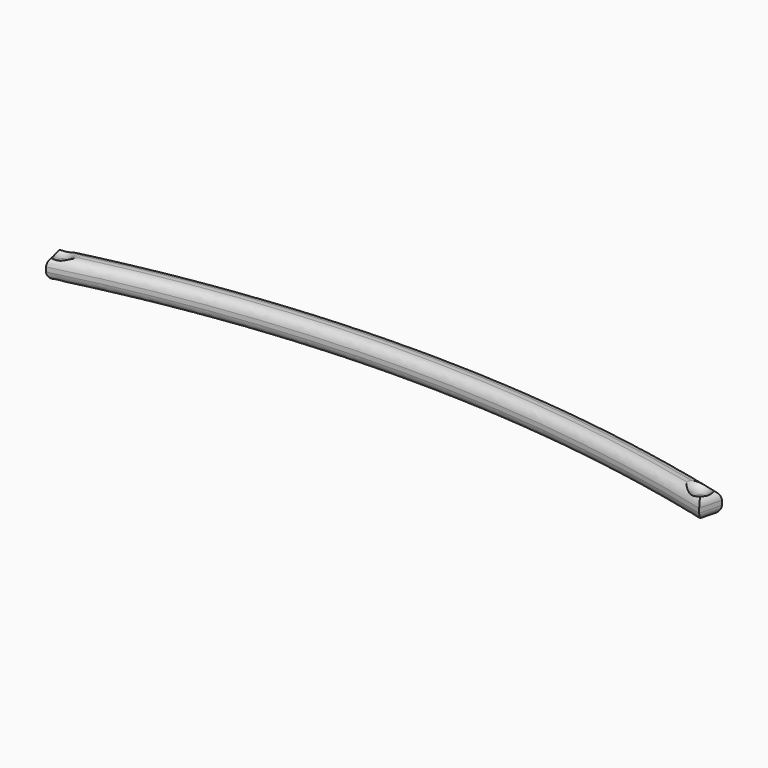
from build123d import *

# Parameters (mm, degrees)
F0_R         = 1.5
F1_DEPTH     = 5
F2_T1_DEPTH  = 15
F2_T3_DEPTH  = 15
F2_T6_ANGLE  = 30.897335
F2_T8_ANGLE  = 30.864963
F2_T14_ANGLE = 30.897335
F2_T16_ANGLE = 30.864963


# Not quite as in the source:
# - a fillet or chamfer that OpenCascade refuses, or shapes differently, is made with other operations: its cross-section is extruded or revolved along the edge and cut away or added


with BuildPart() as f1:
    # F0 (on Top) → F1 (new body)
    with BuildSketch(Plane.XY):
        with BuildLine():
            Line((73.75, -4.841229), (75, 0))
            ThreePointArc((75, 0), (0, 9.526249), (-75, 0))
            Line((-75, 0), (-73.75, -4.841229))
            ThreePointArc((-73.75, -4.841229), (0, 4.526249), (73.75, -4.841229))
        make_face()
        with Locations((-72.566904, -1.807881)):
            Circle(F0_R, mode=Mode.SUBTRACT)
        with Locations((71.612378, -1.807881)):
            Circle(F0_R, mode=Mode.SUBTRACT)
    extrude(amount=F1_DEPTH)

    # F2: fillet of radius 2 on 12 edges, made by hand

    # F2_s2 → F2_t1 (cut)
    with BuildSketch(Plane(origin=(2.1875, 8.472151, 0), x_dir=(0, 0, 1), z_dir=(0.25, 0.968246, 0))):
        with BuildLine():
            ThreePointArc((3, 72.618438), (4.414214, 72.032651), (5, 70.618438))
            Line((5, 70.618438), (5, 72.618438))
            Line((5, 72.618438), (3, 72.618438))
        make_face()
        with BuildLine():
            ThreePointArc((2, 72.618438), (0.585786, 72.032651), (0, 70.618438))
            Line((0, 70.618438), (0, 72.618438))
            Line((0, 72.618438), (2, 72.618438))
        make_face()
    extrude(amount=F2_T1_DEPTH, mode=Mode.SUBTRACT)

    # F2_s4 → F2_t3 (cut)
    with BuildSketch(Plane(origin=(-5.9375, 22.995839, 0), x_dir=(0, 0, 1), z_dir=(0.25, -0.968246, 0))):
        with BuildLine():
            ThreePointArc((3, 72.618438), (4.414214, 72.032651), (5, 70.618438))
            Line((5, 70.618438), (5, 72.618438))
            Line((5, 72.618438), (3, 72.618438))
        make_face()
        with BuildLine():
            ThreePointArc((2, 72.618438), (0.585786, 72.032651), (0, 70.618438))
            Line((0, 70.618438), (0, 72.618438))
            Line((0, 72.618438), (2, 72.618438))
        make_face()
    extrude(amount=F2_T3_DEPTH, mode=Mode.SUBTRACT)

    # F2_s5 → F2_t6 (revolve, cut)
    with BuildSketch(Plane(origin=(-74.57933, -20.61074, 0), x_dir=(0, 0, 1), z_dir=(-0.963869, -0.266375, 0))):
        with BuildLine():
            ThreePointArc((3, 15.021213), (4.414214, 15.607), (5, 17.021213))
            Line((5, 17.021213), (5, 15.021213))
            Line((5, 15.021213), (3, 15.021213))
        make_face()
    revolve(axis=Axis((0, -290.473751, 5), (0, 0, -1)), revolution_arc=F2_T6_ANGLE, mode=Mode.SUBTRACT)

    # F2_s7 → F2_t8 (revolve, cut)
    with BuildSketch(Plane(origin=(74.508905, -20.568623, 0), x_dir=(0, 0, 1), z_dir=(0.963945, -0.266103, 0))):
        with BuildLine():
            ThreePointArc((3, -19.999366), (4.414214, -19.41358), (5, -17.999366))
            Line((5, -17.999366), (5, -19.999366))
            Line((5, -19.999366), (3, -19.999366))
        make_face()
    revolve(axis=Axis((0, -290.473751, 5), (0, 0, 1)), revolution_arc=F2_T8_ANGLE, mode=Mode.SUBTRACT)

    # F2_s9 → F2_t10 (revolve, cut)
    with BuildSketch(Plane.XZ.offset(1.807881)):
        with BuildLine():
            ThreePointArc((-71.066904, 3), (-70.481118, 4.414214), (-69.066904, 5))
            Line((-69.066904, 5), (-71.066904, 5))
            Line((-71.066904, 5), (-71.066904, 3))
        make_face()
    revolve(axis=Axis((-72.566904, -1.807881, 5), (0, 0, 1)), mode=Mode.SUBTRACT)

    # F2_s11 → F2_t12 (revolve, cut)
    with BuildSketch(Plane.XZ.offset(1.807881)):
        with BuildLine():
            ThreePointArc((73.112378, 3), (73.698165, 4.414214), (75.112378, 5))
            Line((75.112378, 5), (73.112378, 5))
            Line((73.112378, 5), (73.112378, 3))
        make_face()
    revolve(axis=Axis((71.612378, -1.807881, 5), (0, 0, 1)), mode=Mode.SUBTRACT)

    # F2_s13 → F2_t14 (revolve, cut)
    with BuildSketch(Plane(origin=(-74.57933, -20.61074, 0), x_dir=(0, 0, 1), z_dir=(-0.963869, -0.266375, 0))):
        with BuildLine():
            ThreePointArc((2, 15.021213), (0.585786, 15.607), (0, 17.021213))
            Line((0, 17.021213), (0, 15.021213))
            Line((0, 15.021213), (2, 15.021213))
        make_face()
    revolve(axis=Axis((0, -290.473751, 0), (0, 0, -1)), revolution_arc=F2_T14_ANGLE, mode=Mode.SUBTRACT)

    # F2_s15 → F2_t16 (revolve, cut)
    with BuildSketch(Plane(origin=(74.508905, -20.568623, 0), x_dir=(0, 0, 1), z_dir=(0.963945, -0.266103, 0))):
        with BuildLine():
            ThreePointArc((2, -19.999366), (0.585786, -19.41358), (0, -17.999366))
            Line((0, -17.999366), (0, -19.999366))
            Line((0, -19.999366), (2, -19.999366))
        make_face()
    revolve(axis=Axis((0, -290.473751, 0), (0, 0, 1)), revolution_arc=F2_T16_ANGLE, mode=Mode.SUBTRACT)

    # F2_s17 → F2_t18 (revolve, cut)
    with BuildSketch(Plane.XZ.offset(1.807881)):
        with BuildLine():
            ThreePointArc((-71.066904, 2), (-70.481118, 0.585786), (-69.066904, 0))
            Line((-69.066904, 0), (-71.066904, 0))
            Line((-71.066904, 0), (-71.066904, 2))
        make_face()
    revolve(axis=Axis((-72.566904, -1.807881, 0), (0, 0, 1)), mode=Mode.SUBTRACT)

    # F2_s19 → F2_t20 (revolve, cut)
    with BuildSketch(Plane.XZ.offset(1.807881)):
        with BuildLine():
            ThreePointArc((73.112378, 2), (73.698165, 0.585786), (75.112378, 0))
            Line((75.112378, 0), (73.112378, 0))
            Line((73.112378, 0), (73.112378, 2))
        make_face()
    revolve(axis=Axis((71.612378, -1.807881, 0), (0, 0, 1)), mode=Mode.SUBTRACT)


solid = f1.part
